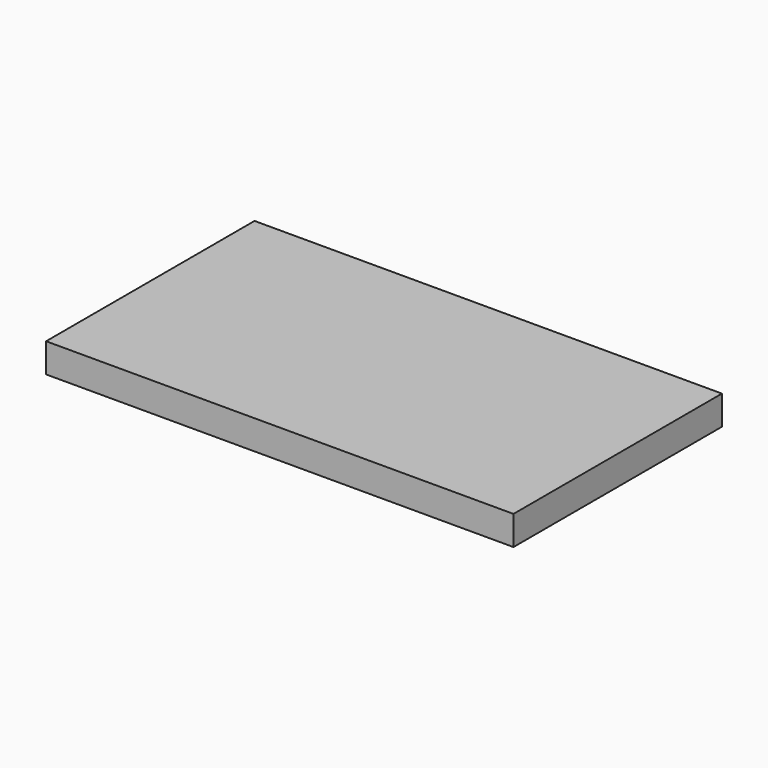
from build123d import *

# Parameters (mm, degrees)
F0_W     = 101.618539542
F0_H     = 56.6494166851
F1_DEPTH = 6.35


# Not quite as in the source:
# - the program builds the solid bodies; features that only make, move or delete a surface that nothing else refers to are left out


with BuildPart() as f1:
    # F0 (on Top) → F1 (new body)
    with BuildSketch(Plane.XY):
        with Locations((-1.8626e-06, 1.4600362629)):
            Rectangle(F0_W, F0_H)
    extrude(amount=F1_DEPTH)


solid = f1.part
